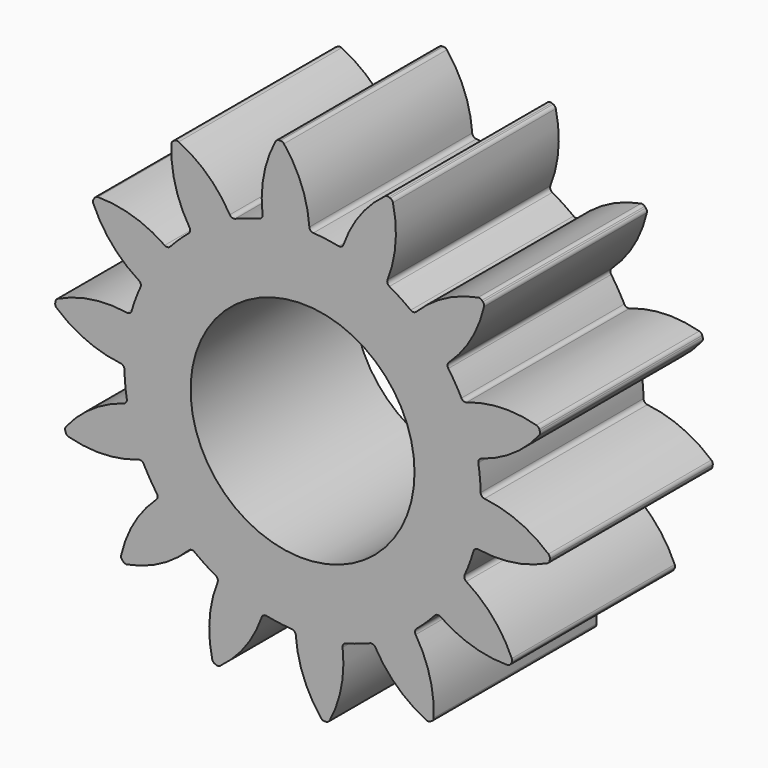
from build123d import *

# Parameters (mm, degrees)
F1_DEPTH = 2
F2_R     = 1.1
F3_DEPTH = 2.001


# Not quite as in the source:
# - a feature names something its author has since deleted; it is built from what else it names


with BuildPart() as f1:
    # F0 (on Front) → F1 (new body)
    with BuildSketch(Plane.XZ):
        with BuildLine():
            ThreePointArc((0.0666269178, 1.7858202042), (-0.0091119072, 2.1241856215), (-0.1822631738, 2.4245956149))
            ThreePointArc((-0.1822631738, 2.4245956149), (-0.1985798387, 2.4370017758), (-0.2188249812, 2.4402081115))
            ThreePointArc((-0.2188249812, 2.4402081115), (-0.2260574807, 2.4395487319), (-0.2332879938, 2.4388679161))
            ThreePointArc((-0.2332879938, 2.4388679161), (-0.2525992616, 2.4319961391), (-0.2663584782, 2.4168030373))
            ThreePointArc((-0.2663584782, 2.4168030373), (-0.381361324, 2.0896916332), (-0.3936360694, 1.7431705575))
            ThreePointArc((-0.3936360694, 1.7431705575), (-0.400802791, 1.7144337142), (-0.425150562, 1.6975709115))
            ThreePointArc((-0.425150562, 1.6975709115), (-0.5451717214, 1.6629154501), (-0.6624147605, 1.6197859998))
            ThreePointArc((-0.6624147605, 1.6197859998), (-0.9015366272, 1.4999105673), (-1.119595835, 1.3449926268))
            ThreePointArc((-1.119595835, 1.3449926268), (-1.212694722, 1.2616939056), (-1.299613883, 1.1719657653))
            ThreePointArc((-1.299613883, 1.1719657653), (-1.4630432396, 0.960210643), (-1.592291422, 0.7260220571))
            ThreePointArc((-1.592291422, 0.7260220571), (-1.6400286601, 0.6105784094), (-1.6794085373, 0.4920233378))
            ThreePointArc((-1.6794085373, 0.4920233378), (-1.7347761954, 0.2303292247), (-1.7496141647, -0.0367460851))
            ThreePointArc((-1.7496141647, -0.0367460851), (-1.7425348085, -0.1614696291), (-1.7265757341, -0.285370346))
            ThreePointArc((-1.7265757341, -0.285370346), (-1.6629154501, -0.5451717214), (-1.5604043644, -0.7922362145))
            ThreePointArc((-1.5604043644, -0.7922362145), (-1.4999105673, -0.9015366272), (-1.4317734318, -1.0062429329))
            ThreePointArc((-1.4317734318, -1.0062429329), (-1.2616939056, -1.212694722), (-1.0621373427, -1.3908142454))
            ThreePointArc((-1.0621373427, -1.3908142454), (-0.960210643, -1.4630432396), (-0.8533908417, -1.5278167663))
            ThreePointArc((-0.8533908417, -1.5278167663), (-0.6105784094, -1.6400286601), (-0.353500994, -1.7139244579))
            ThreePointArc((-0.353500994, -1.7139244579), (-0.2303292247, -1.7347761954), (-0.1059837293, -1.7467877516))
            ThreePointArc((-0.1059837293, -1.7467877516), (0.1614696291, -1.7425348085), (0.425150562, -1.6975709115))
            ThreePointArc((0.425150562, -1.6975709115), (0.5451717214, -1.6629154501), (0.6624147605, -1.6197859998))
            ThreePointArc((0.6624147605, -1.6197859998), (0.9015366272, -1.4999105673), (1.119595835, -1.3449926268))
            ThreePointArc((1.119595835, -1.3449926268), (1.212694722, -1.2616939056), (1.299613883, -1.1719657653))
            ThreePointArc((1.299613883, -1.1719657653), (1.4630432396, -0.960210643), (1.592291422, -0.7260220571))
            ThreePointArc((1.592291422, -0.7260220571), (1.6400286601, -0.6105784094), (1.6794085373, -0.4920233378))
            ThreePointArc((1.6794085373, -0.4920233378), (1.7347761954, -0.2303292247), (1.7496141647, 0.0367460851))
            ThreePointArc((1.7496141647, 0.0367460851), (1.7425348085, 0.1614696291), (1.7265757341, 0.285370346))
            ThreePointArc((1.7265757341, 0.285370346), (1.6629154501, 0.5451717214), (1.5604043644, 0.7922362145))
            ThreePointArc((1.5604043644, 0.7922362145), (1.4999105673, 0.9015366272), (1.4317734318, 1.0062429329))
            ThreePointArc((1.4317734318, 1.0062429329), (1.2616939056, 1.212694722), (1.0621373427, 1.3908142454))
            ThreePointArc((1.0621373427, 1.3908142454), (0.960210643, 1.4630432396), (0.8533908417, 1.5278167663))
            ThreePointArc((0.8533908417, 1.5278167663), (0.6105784094, 1.6400286601), (0.353500994, 1.7139244579))
            ThreePointArc((0.353500994, 1.7139244579), (0.2303292247, 1.7347761954), (0.1059837293, 1.7467877516))
            ThreePointArc((0.1059837293, 1.7467877516), (0.0789519935, 1.7588895418), (0.0666269178, 1.7858202042))
        make_face()
        with BuildLine():
            ThreePointArc((-1.119595835, 1.3449926268), (-0.9015366272, 1.4999105673), (-0.6624147605, 1.6197859998))
            ThreePointArc((-0.6624147605, 1.6197859998), (-0.6920202829, 1.6189607054), (-0.7148095688, 1.6378767438))
            ThreePointArc((-0.7148095688, 1.6378767438), (-0.9298591447, 1.9098716062), (-1.2162060566, 2.1054041389))
            ThreePointArc((-1.2162060566, 2.1054041389), (-1.2362896952, 2.109502168), (-1.2559211152, 2.1036069386))
            ThreePointArc((-1.2559211152, 2.1036069386), (-1.262151278, 2.0998747942), (-1.2683703503, 2.0961241982))
            ThreePointArc((-1.2683703503, 2.0961241982), (-1.2827876491, 2.081554096), (-1.2885922351, 2.061895684))
            ThreePointArc((-1.2885922351, 2.061895684), (-1.2502778998, 1.7172806278), (-1.1109872032, 1.3997501142))
            ThreePointArc((-1.1109872032, 1.3997501142), (-1.1049757472, 1.3707495889), (-1.119595835, 1.3449926268))
        make_face()
        with BuildLine():
            ThreePointArc((-1.592291422, 0.7260220571), (-1.4630432396, 0.960210643), (-1.299613883, 1.1719657653))
            ThreePointArc((-1.299613883, 1.1719657653), (-1.3259294552, 1.158376846), (-1.3546692538, 1.1655317072))
            ThreePointArc((-1.3546692538, 1.1655317072), (-1.6664363747, 1.3172840963), (-2.0092644141, 1.3692115521))
            ThreePointArc((-2.0092644141, 1.3692115521), (-2.0291372154, 1.3641897846), (-2.0442666695, 1.3503606125))
            ThreePointArc((-2.0442666695, 1.3503606125), (-2.0482605355, 1.3442949002), (-2.0522364034, 1.3382173757))
            ThreePointArc((-2.0522364034, 1.3382173757), (-2.0589042103, 1.3188347357), (-2.0556044963, 1.298604603))
            ThreePointArc((-2.0556044963, 1.298604603), (-1.8715616038, 1.004741133), (-1.6082936961, 0.7790919939))
            ThreePointArc((-1.6082936961, 0.7790919939), (-1.5902947051, 0.7555716965), (-1.592291422, 0.7260220571))
        make_face()
        with BuildLine():
            ThreePointArc((-1.7496141647, -0.0367460851), (-1.7347761954, 0.2303292247), (-1.6794085373, 0.4920233378))
            ThreePointArc((-1.6794085373, 0.4920233378), (-1.6972220374, 0.4683622458), (-1.7262200792, 0.4623388216))
            ThreePointArc((-1.7262200792, 0.4623388216), (-2.0729554431, 0.4637923157), (-2.4043633124, 0.3618298252))
            ThreePointArc((-2.4043633124, 0.3618298252), (-2.4200892244, 0.3486828836), (-2.4277201387, 0.329658806))
            ThreePointArc((-2.4277201387, 0.329658806), (-2.4286866736, 0.3224609146), (-2.4296318677, 0.3152601897))
            ThreePointArc((-2.4296318677, 0.3152601897), (-2.4272295419, 0.2949039815), (-2.4154790767, 0.278108954))
            ThreePointArc((-2.4154790767, 0.278108954), (-2.1221595791, 0.0932003345), (-1.787057898, 0.0041251493))
            ThreePointArc((-1.787057898, 0.0041251493), (-1.7606362929, -0.0092564369), (-1.7496141647, -0.0367460851))
        make_face()
        with BuildLine():
            ThreePointArc((-1.5604043644, -0.7922362145), (-1.6629154501, -0.5451717214), (-1.7265757341, -0.285370346))
            ThreePointArc((-1.7265757341, -0.285370346), (-1.7323589801, -0.3144172414), (-1.7558718472, -0.3324259378))
            ThreePointArc((-1.7558718472, -0.3324259378), (-2.0689002629, -0.4815592211), (-2.323248569, -0.7172167362))
            ThreePointArc((-2.323248569, -0.7172167362), (-2.331712882, -0.7358849388), (-2.3303338603, -0.7563359701))
            ThreePointArc((-2.3303338603, -0.7563359701), (-2.3280816301, -0.7632404099), (-2.3258089432, -0.7701381432))
            ThreePointArc((-2.3258089432, -0.7701381432), (-2.3148122947, -0.787436123), (-2.296938402, -0.7974695841))
            ThreePointArc((-2.296938402, -0.7974695841), (-1.9524378231, -0.8367999333), (-1.6118733664, -0.7716587318))
            ThreePointArc((-1.6118733664, -0.7716587318), (-1.5822622701, -0.7722512195), (-1.5604043644, -0.7922362145))
        make_face()
        with BuildLine():
            ThreePointArc((0.4016795156, 1.7413346934), (0.3827540735, 1.7185532161), (0.353500994, 1.7139244579))
            ThreePointArc((0.353500994, 1.7139244579), (0.6105784094, 1.6400286601), (0.8533908417, 1.5278167663))
            ThreePointArc((0.8533908417, 1.5278167663), (0.8342868593, 1.5504487331), (0.8348671263, 1.5800600714))
            ThreePointArc((0.8348671263, 1.5800600714), (0.9134400553, 1.917778623), (0.8877791659, 2.2635661936))
            ThreePointArc((0.8877791659, 2.2635661936), (0.8784611902, 2.2818232939), (0.8616121241, 2.2934961407))
            ThreePointArc((0.8616121241, 2.2934961407), (0.8548097731, 2.2960401242), (0.8479999109, 2.2985639323))
            ThreePointArc((0.8479999109, 2.2985639323), (0.8276195076, 2.3007515203), (0.808630842, 2.293032909))
            ThreePointArc((0.808630842, 2.293032909), (0.563088539, 2.0482135823), (0.4016795156, 1.7413346934))
        make_face()
        with BuildLine():
            ThreePointArc((1.1174375463, 1.3946061372), (1.0905017996, 1.382292177), (1.0621373427, 1.3908142454))
            ThreePointArc((1.0621373427, 1.3908142454), (1.2616939056, 1.212694722), (1.4317734318, 1.0062429329))
            ThreePointArc((1.4317734318, 1.0062429329), (1.4243809807, 1.0349225378), (1.4377516614, 1.0613496633))
            ThreePointArc((1.4377516614, 1.0613496633), (1.6550740123, 1.3315320482), (1.7819859538, 1.6542097269))
            ThreePointArc((1.7819859538, 1.6542097269), (1.7815122068, 1.674701724), (1.7713963812, 1.6925291314))
            ThreePointArc((1.7713963812, 1.6925291314), (1.7663714678, 1.6977726107), (1.7613310333, 1.7030011718))
            ThreePointArc((1.7613310333, 1.7030011718), (1.7439180832, 1.713814846), (1.7234609067, 1.7150994908))
            ThreePointArc((1.7234609067, 1.7150994908), (1.3960118111, 1.6010617117), (1.1174375463, 1.3946061372))
        make_face()
        with BuildLine():
            ThreePointArc((1.6118733664, 0.7716587318), (1.5822622701, 0.7722512195), (1.5604043644, 0.7922362145))
            ThreePointArc((1.5604043644, 0.7922362145), (1.6629154501, 0.5451717214), (1.7265757341, 0.285370346))
            ThreePointArc((1.7265757341, 0.285370346), (1.7323589801, 0.3144172414), (1.7558718472, 0.3324259378))
            ThreePointArc((1.7558718472, 0.3324259378), (2.0689002629, 0.4815592211), (2.323248569, 0.7172167362))
            ThreePointArc((2.323248569, 0.7172167362), (2.331712882, 0.7358849388), (2.3303338603, 0.7563359701))
            ThreePointArc((2.3303338603, 0.7563359701), (2.3280816301, 0.7632404099), (2.3258089432, 0.7701381432))
            ThreePointArc((2.3258089432, 0.7701381432), (2.3148122947, 0.787436123), (2.296938402, 0.7974695841))
            ThreePointArc((2.296938402, 0.7974695841), (1.9524378231, 0.8367999333), (1.6118733664, 0.7716587318))
        make_face()
        with BuildLine():
            ThreePointArc((1.787057898, -0.0041251493), (1.7606362929, 0.0092564369), (1.7496141647, 0.0367460851))
            ThreePointArc((1.7496141647, 0.0367460851), (1.7347761954, -0.2303292247), (1.6794085373, -0.4920233378))
            ThreePointArc((1.6794085373, -0.4920233378), (1.6972220374, -0.4683622458), (1.7262200792, -0.4623388216))
            ThreePointArc((1.7262200792, -0.4623388216), (2.0729554431, -0.4637923157), (2.4043633124, -0.3618298252))
            ThreePointArc((2.4043633124, -0.3618298252), (2.4200892244, -0.3486828836), (2.4277201387, -0.329658806))
            ThreePointArc((2.4277201387, -0.329658806), (2.4286866736, -0.3224609146), (2.4296318677, -0.3152601897))
            ThreePointArc((2.4296318677, -0.3152601897), (2.4272295419, -0.2949039815), (2.4154790767, -0.278108954))
            ThreePointArc((2.4154790767, -0.278108954), (2.1221595791, -0.0932003345), (1.787057898, -0.0041251493))
        make_face()
        with BuildLine():
            ThreePointArc((1.6082936961, -0.7790919939), (1.5902947051, -0.7555716965), (1.592291422, -0.7260220571))
            ThreePointArc((1.592291422, -0.7260220571), (1.4630432396, -0.960210643), (1.299613883, -1.1719657653))
            ThreePointArc((1.299613883, -1.1719657653), (1.3259294552, -1.158376846), (1.3546692538, -1.1655317072))
            ThreePointArc((1.3546692538, -1.1655317072), (1.6664363747, -1.3172840963), (2.0092644141, -1.3692115521))
            ThreePointArc((2.0092644141, -1.3692115521), (2.0291372154, -1.3641897846), (2.0442666695, -1.3503606125))
            ThreePointArc((2.0442666695, -1.3503606125), (2.0482605355, -1.3442949002), (2.0522364034, -1.3382173757))
            ThreePointArc((2.0522364034, -1.3382173757), (2.0589042103, -1.3188347357), (2.0556044963, -1.298604603))
            ThreePointArc((2.0556044963, -1.298604603), (1.8715616038, -1.004741133), (1.6082936961, -0.7790919939))
        make_face()
        with BuildLine():
            ThreePointArc((1.1109872032, -1.3997501142), (1.1049757472, -1.3707495889), (1.119595835, -1.3449926268))
            ThreePointArc((1.119595835, -1.3449926268), (0.9015366272, -1.4999105673), (0.6624147605, -1.6197859998))
            ThreePointArc((0.6624147605, -1.6197859998), (0.6920202829, -1.6189607054), (0.7148095688, -1.6378767438))
            ThreePointArc((0.7148095688, -1.6378767438), (0.9298591447, -1.9098716062), (1.2162060566, -2.1054041389))
            ThreePointArc((1.2162060566, -2.1054041389), (1.2362896952, -2.109502168), (1.2559211152, -2.1036069386))
            ThreePointArc((1.2559211152, -2.1036069386), (1.262151278, -2.0998747942), (1.2683703503, -2.0961241982))
            ThreePointArc((1.2683703503, -2.0961241982), (1.2827876491, -2.081554096), (1.2885922351, -2.061895684))
            ThreePointArc((1.2885922351, -2.061895684), (1.2502778998, -1.7172806278), (1.1109872032, -1.3997501142))
        make_face()
        with BuildLine():
            ThreePointArc((0.3936360694, -1.7431705575), (0.400802791, -1.7144337142), (0.425150562, -1.6975709115))
            ThreePointArc((0.425150562, -1.6975709115), (0.1614696291, -1.7425348085), (-0.1059837293, -1.7467877516))
            ThreePointArc((-0.1059837293, -1.7467877516), (-0.0789519935, -1.7588895418), (-0.0666269178, -1.7858202042))
            ThreePointArc((-0.0666269178, -1.7858202042), (0.0091119072, -2.1241856215), (0.1822631738, -2.4245956149))
            ThreePointArc((0.1822631738, -2.4245956149), (0.1985798387, -2.4370017758), (0.2188249812, -2.4402081115))
            ThreePointArc((0.2188249812, -2.4402081115), (0.2260574807, -2.4395487319), (0.2332879938, -2.4388679161))
            ThreePointArc((0.2332879938, -2.4388679161), (0.2525992616, -2.4319961391), (0.2663584782, -2.4168030373))
            ThreePointArc((0.2663584782, -2.4168030373), (0.381361324, -2.0896916332), (0.3936360694, -1.7431705575))
        make_face()
        with BuildLine():
            ThreePointArc((-0.353500994, -1.7139244579), (-0.6105784094, -1.6400286601), (-0.8533908417, -1.5278167663))
            ThreePointArc((-0.8533908417, -1.5278167663), (-0.8342868593, -1.5504487331), (-0.8348671263, -1.5800600714))
            ThreePointArc((-0.8348671263, -1.5800600714), (-0.9134400553, -1.917778623), (-0.8877791659, -2.2635661936))
            ThreePointArc((-0.8877791659, -2.2635661936), (-0.8784611902, -2.2818232939), (-0.8616121241, -2.2934961407))
            ThreePointArc((-0.8616121241, -2.2934961407), (-0.8548097731, -2.2960401242), (-0.8479999109, -2.2985639323))
            ThreePointArc((-0.8479999109, -2.2985639323), (-0.8276195076, -2.3007515203), (-0.808630842, -2.293032909))
            ThreePointArc((-0.808630842, -2.293032909), (-0.563088539, -2.0482135823), (-0.4016795156, -1.7413346934))
            ThreePointArc((-0.4016795156, -1.7413346934), (-0.3827540735, -1.7185532161), (-0.353500994, -1.7139244579))
        make_face()
        with BuildLine():
            ThreePointArc((-1.0621373427, -1.3908142454), (-1.2616939056, -1.212694722), (-1.4317734318, -1.0062429329))
            ThreePointArc((-1.4317734318, -1.0062429329), (-1.4243809807, -1.0349225378), (-1.4377516614, -1.0613496633))
            ThreePointArc((-1.4377516614, -1.0613496633), (-1.6550740123, -1.3315320482), (-1.7819859538, -1.6542097269))
            ThreePointArc((-1.7819859538, -1.6542097269), (-1.7815122068, -1.674701724), (-1.7713963812, -1.6925291314))
            ThreePointArc((-1.7713963812, -1.6925291314), (-1.7663714678, -1.6977726107), (-1.7613310333, -1.7030011718))
            ThreePointArc((-1.7613310333, -1.7030011718), (-1.7439180832, -1.713814846), (-1.7234609067, -1.7150994908))
            ThreePointArc((-1.7234609067, -1.7150994908), (-1.3960118111, -1.6010617117), (-1.1174375463, -1.3946061372))
            ThreePointArc((-1.1174375463, -1.3946061372), (-1.0905017996, -1.382292177), (-1.0621373427, -1.3908142454))
        make_face()
    extrude(amount=F1_DEPTH)

    # F2 (on face) → F3 (cut, through all)
    with BuildSketch(Plane.XZ.offset(2)):
        Circle(F2_R)
    extrude(amount=-F3_DEPTH, mode=Mode.SUBTRACT)


solid = f1.part
